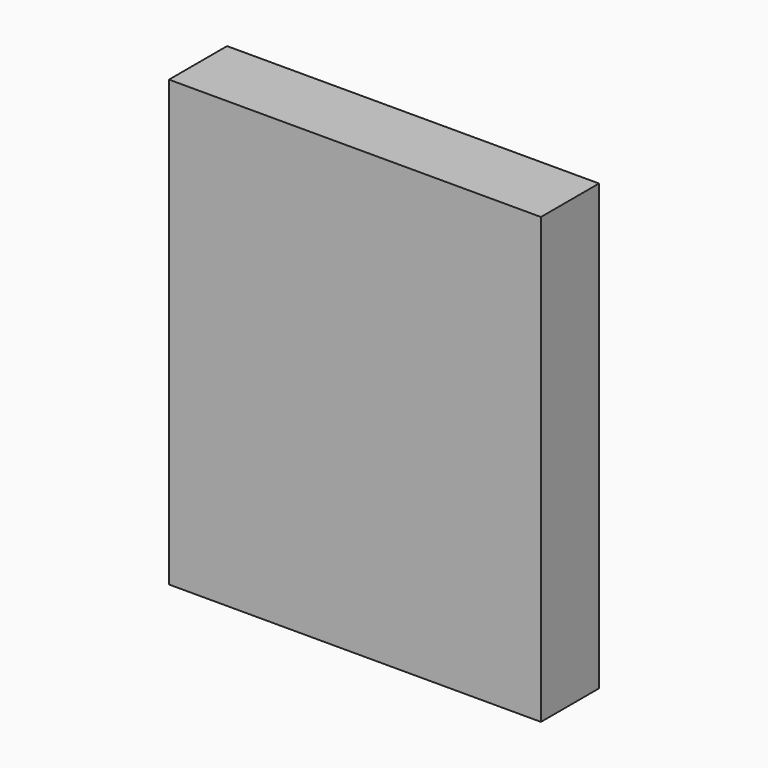
from build123d import *

# Parameters (mm, degrees)
F0_W     = 41
F0_H     = 49
F1_DEPTH = 8
F3_DEPTH = 1
F4_SIZE2 = 2.99999
F4_SIZE  = 0.99999


# Not quite as in the source:
# - a fillet or chamfer is up to 0.001 mm smaller than in the source, because OpenCascade refuses the exact size


with BuildPart() as f1:
    # F0 (on Front) → F1 (new body)
    with BuildSketch(Plane.XZ):
        Rectangle(F0_W, F0_H)
    extrude(amount=F1_DEPTH)

    # F2 (on Front) → F3 (cut)
    with BuildSketch(Plane.XZ):
        with BuildLine():
            Line((3, 20), (-3, 20))
            ThreePointArc((-3, 20), (0, 17), (3, 20))
        make_face()
    extrude(amount=F3_DEPTH, mode=Mode.SUBTRACT)

    # F4 (size 1 and 3 in the source; OpenCascade refuses exactly that, so slightly less here)
    f4_edges = [f1.edges().sort_by_distance(p)[0] for p in [
        (0, -1, 20),
    ]]
    chamfer(f4_edges, length=F4_SIZE, length2=F4_SIZE2)


solid = f1.part
